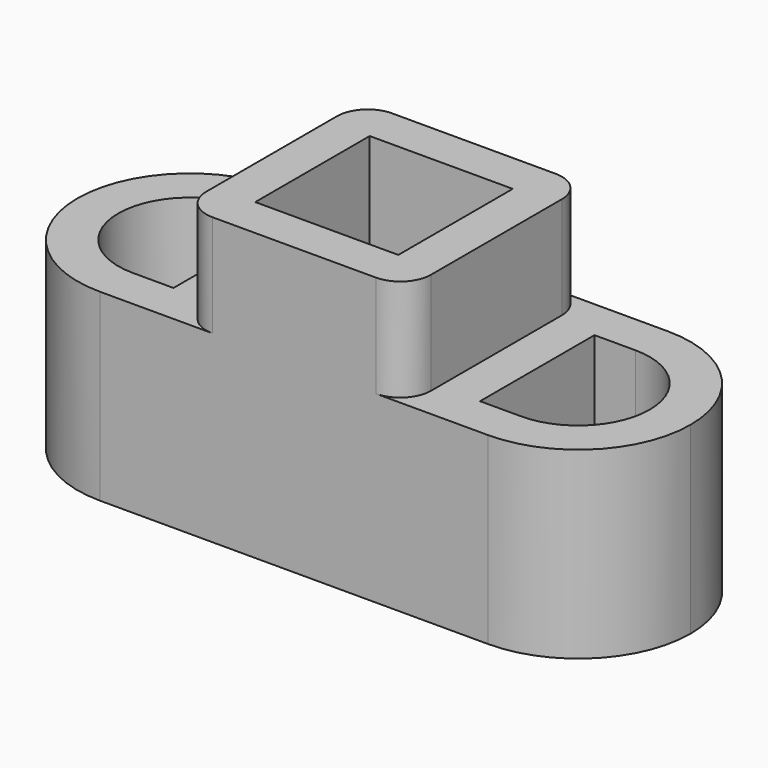
from build123d import *

# Parameters (mm, degrees)
F0_W     = 30
F0_H     = 11
F1_DEPTH = 9
F2_W     = 11
F2_H     = 11
F3_DEPTH = 5
F4_R     = 1.5
F5_R     = 5.49999
F6_W     = 7
F6_H     = 7
F7_DEPTH = 25
F9_DEPTH = 25


# Not quite as in the source:
# - a fillet or chamfer is up to 0.001 mm smaller than in the source, because OpenCascade refuses the exact size


with BuildPart() as f1:
    # F0 (on Top) → F1 (new body)
    with BuildSketch(Plane.XY):
        with Locations((15, 5.5)):
            Rectangle(F0_W, F0_H)
    extrude(amount=F1_DEPTH)

    # F2 (on face) → F3 (join)
    with BuildSketch(Plane.XY.offset(9)):
        with Locations((15, 5.5)):
            Rectangle(F2_W, F2_H)
    extrude(amount=F3_DEPTH)

    # F4
    f4_edges = [f1.edges().sort_by_distance(p)[0] for p in [
        (20.5, 11, 11.5),
        (9.5, 11, 11.5),
        (9.5, 0, 11.5),
        (20.5, 0, 11.5),
    ]]
    fillet(f4_edges, radius=F4_R)

    # F5 (radius 5.5 in the source; OpenCascade refuses exactly that, so slightly less here)
    f5_edges = [f1.edges().sort_by_distance(p)[0] for p in [
        (30, 11, 4.5),
        (30, 0, 4.5),
        (0, 11, 4.5),
        (0, 0, 4.5),
    ]]
    fillet(f5_edges, radius=F5_R)

    # F6 (on face) → F7 (cut)
    with BuildSketch(Plane.XY.offset(14)):
        with Locations((15, 5.5)):
            Rectangle(F6_W, F6_H)
    extrude(amount=-F7_DEPTH, mode=Mode.SUBTRACT)

    # F8 (on face) → F9 (cut)
    with BuildSketch(Plane.XY.offset(9)):
        with BuildLine():
            Line((24.5, 9), (22.5, 9))
            Line((22.5, 9), (22.5, 2))
            Line((22.5, 2), (24.5, 2))
            ThreePointArc((24.5, 2), (28, 5.5), (24.5, 9))
        make_face()
        with BuildLine():
            Line((7.5, 2), (7.5, 9))
            Line((7.5, 9), (5.5, 9))
            ThreePointArc((5.5, 9), (2, 5.5), (5.5, 2))
            Line((5.5, 2), (7.5, 2))
        make_face()
    extrude(amount=-F9_DEPTH, mode=Mode.SUBTRACT)


solid = f1.part
